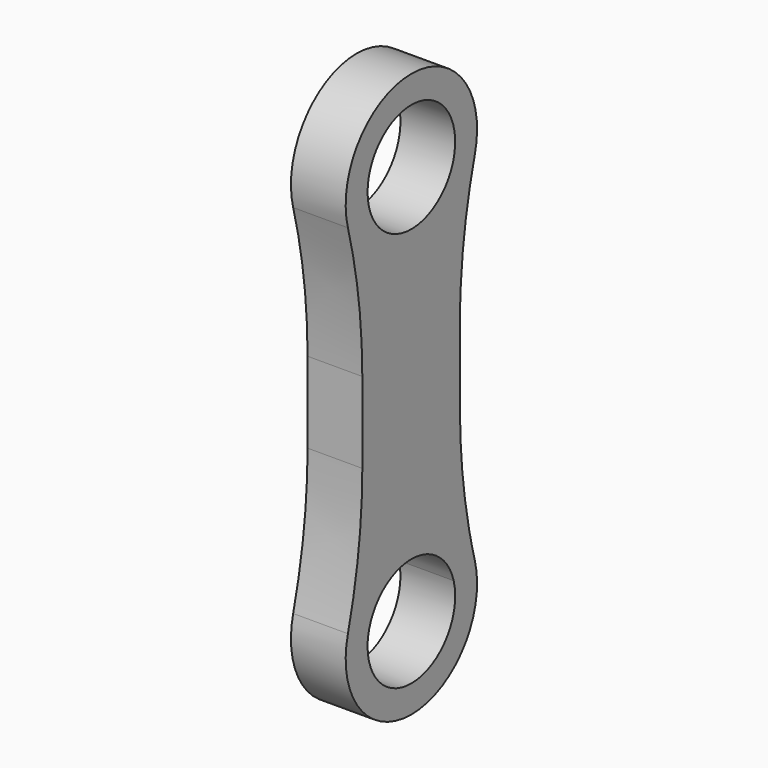
from build123d import *

# Parameters (mm, degrees)
F2_W          = 56.6284824163
F2_H          = 136.3001726568
F3_DEPTH      = 25.4
F0_R          = 38.1
F4_DEPTH      = 25.4
F1_R          = 38.1
F5_DEPTH      = 25.4
F6_D          = 50.8
F8_D          = 50.8
F11_T4_DEPTH  = 25.4
F11_S5_R      = 25.4
F11_T6_DEPTH  = 43
F11_T10_DEPTH = 25.4
F11_S11_R     = 25.4
F11_T12_DEPTH = 43
F11_T16_DEPTH = 25.4
F11_S17_R     = 25.4
F11_T18_DEPTH = 43
F11_T22_DEPTH = 25.4
F11_S23_R     = 25.4
F11_T24_DEPTH = 43


# Not quite as in the source:
# - a fillet or chamfer that OpenCascade refuses, or shapes differently, is made with other operations: its cross-section is extruded or revolved along the edge and cut away or added
# - two fillets or chamfers of one size are made in one step


with BuildPart() as f3:
    # F2 (on Right) → F3 (new body)
    with BuildSketch(Plane.YZ):
        with Locations((-0.1386040822, -92.7020926028)):
            Rectangle(F2_W, F2_H)
    extrude(amount=F3_DEPTH)

    # F0 (on Right) → F4 (join)
    with BuildSketch(Plane.YZ):
        Circle(F0_R)
    extrude(amount=F4_DEPTH)

    # F1 (on Right) → F5 (join)
    with BuildSketch(Plane.YZ):
        with Locations((0, -185.5300813913)):
            Circle(F1_R)
    extrude(amount=F5_DEPTH)

    # F6 (through all)
    with Locations(Plane(origin=(0, 0, 0), x_dir=(0, 1, 0), z_dir=(-1, 0, 0))):
        with Locations((0, 0)):
            Hole(F6_D / 2)

    # F8 (through all)
    with Locations(Plane.YZ.offset(25.4)):
        with Locations((0, -185.5300813913)):
            Hole(F8_D / 2)

    # F11: fillet of radius 254 on 4 edges, made by hand


with BuildPart() as f11_tool2:
    # F11_s3 → F11_t4 (new body)
    with BuildSketch(Plane.YZ.offset(25.4)):
        with BuildLine():
            add(Edge.make_bspline(
                [(-28.4524452903, -111.0798377649), (-28.4524452903, -143.9931007722), (-36.841297299, -175.8193484896)],
                knots=[0, 0, 0, 1, 1, 1], degree=2, weights=[1, 1, 1]))
            Line((-36.841297299, -175.8193484896), (-12.2799424998, -182.293299562))
            ThreePointArc((-12.2799424998, -182.293299562), (-11.1895620368, -179.5236177494), (-9.4841025329, -177.0840347894))
            Line((-9.4841025329, -177.0840347894), (-3.0526052903, -160.1914627454))
            ThreePointArc((-3.0526052903, -160.1914627454), (-3.0526052903, -135.6356502551), (-3.0522052903, -111.0798377649))
            Line((-3.0522052903, -111.0798377649), (-28.4524452903, -111.0798377649))
        make_face()
    extrude(amount=-F11_T4_DEPTH)

    # F11_s5 → F11_t6 (cut, symmetric)
    with BuildSketch(Plane.YZ.offset(12.7)):
        with Locations((0, -185.5300813913)):
            Circle(F11_S5_R)
    extrude(amount=F11_T6_DEPTH, both=True, mode=Mode.SUBTRACT)


with BuildPart() as f3_1:
    add(f3.part)

    # F11_t1: union F11_tool2
    add(f11_tool2.part)


with BuildPart() as f11_tool8:
    # F11_s9 → F11_t10 (new body)
    with BuildSketch(Plane.YZ.offset(25.4)):
        with BuildLine():
            add(Edge.make_bspline(
                [(-36.841297299, -9.7107329018), (-28.4524452903, -41.5369806191), (-28.4524452903, -74.4502436264)],
                knots=[0, 0, 0, 1, 1, 1], degree=2, weights=[1, 1, 1]))
            Line((-28.4524452903, -74.4502436264), (-3.0522052903, -74.4502436264))
            ThreePointArc((-3.0522052903, -74.4502436264), (-3.0526052903, -49.8944311362), (-3.0526052903, -25.338618646))
            Line((-3.0526052903, -25.338618646), (-9.4841025329, -8.446046602))
            ThreePointArc((-9.4841025329, -8.446046602), (-11.1895620368, -6.0064636419), (-12.2799424998, -3.2367818293))
            Line((-12.2799424998, -3.2367818293), (-36.841297299, -9.7107329018))
        make_face()
    extrude(amount=-F11_T10_DEPTH)

    # F11_s11 → F11_t12 (cut, symmetric)
    with BuildSketch(Plane.YZ.offset(12.7)):
        Circle(F11_S11_R)
    extrude(amount=F11_T12_DEPTH, both=True, mode=Mode.SUBTRACT)


with BuildPart() as f3_2:
    add(f3_1.part)

    # F11_t7: union F11_tool8
    add(f11_tool8.part)


with BuildPart() as f11_tool14:
    # F11_s15 → F11_t16 (new body)
    with BuildSketch(Plane.YZ.offset(25.4)):
        with BuildLine():
            add(Edge.make_bspline(
                [(36.8051403395, -9.8468860434), (28.175237126, -42.1032559751), (28.175237126, -75.4941024849)],
                knots=[0, 0, 0, 1, 1, 1], degree=2, weights=[1, 1, 1]))
            Line((28.175237126, -75.4941024849), (2.774997126, -75.4941024849))
            ThreePointArc((2.774997126, -75.4941024849), (2.775397126, -50.5703062168), (2.775397126, -25.6465099486))
            Line((2.775397126, -25.6465099486), (9.3917015577, -8.5486750967))
            ThreePointArc((9.3917015577, -8.5486750967), (11.1455038849, -6.0878277907), (12.2678906608, -3.2821643992))
            Line((12.2678906608, -3.2821643992), (36.8051403395, -9.8468860434))
        make_face()
    extrude(amount=-F11_T16_DEPTH)

    # F11_s17 → F11_t18 (cut, symmetric)
    with BuildSketch(Plane.YZ.offset(12.7)):
        Circle(F11_S17_R)
    extrude(amount=F11_T18_DEPTH, both=True, mode=Mode.SUBTRACT)


with BuildPart() as f3_3:
    add(f3_2.part)

    # F11_t13: union F11_tool14
    add(f11_tool14.part)


with BuildPart() as f11_tool20:
    # F11_s21 → F11_t22 (new body)
    with BuildSketch(Plane.YZ.offset(25.4)):
        with BuildLine():
            add(Edge.make_bspline(
                [(28.175237126, -110.0359789064), (28.175237126, -143.4268254163), (36.8051403395, -175.683195348)],
                knots=[0, 0, 0, 1, 1, 1], degree=2, weights=[1, 1, 1]))
            Line((36.8051403395, -175.683195348), (12.2678906608, -182.2479169921))
            ThreePointArc((12.2678906608, -182.2479169921), (11.1455038849, -179.4422536006), (9.3917015577, -176.9814062946))
            Line((9.3917015577, -176.9814062946), (2.775397126, -159.8835714427))
            ThreePointArc((2.775397126, -159.8835714427), (2.775397126, -134.9597751745), (2.774997126, -110.0359789064))
            Line((2.774997126, -110.0359789064), (28.175237126, -110.0359789064))
        make_face()
    extrude(amount=-F11_T22_DEPTH)

    # F11_s23 → F11_t24 (cut, symmetric)
    with BuildSketch(Plane.YZ.offset(12.7)):
        with Locations((0, -185.5300813913)):
            Circle(F11_S23_R)
    extrude(amount=F11_T24_DEPTH, both=True, mode=Mode.SUBTRACT)


with BuildPart() as f3_4:
    add(f3_3.part)

    # F11_t19: union F11_tool20
    add(f11_tool20.part)


solid = f3_4.part
